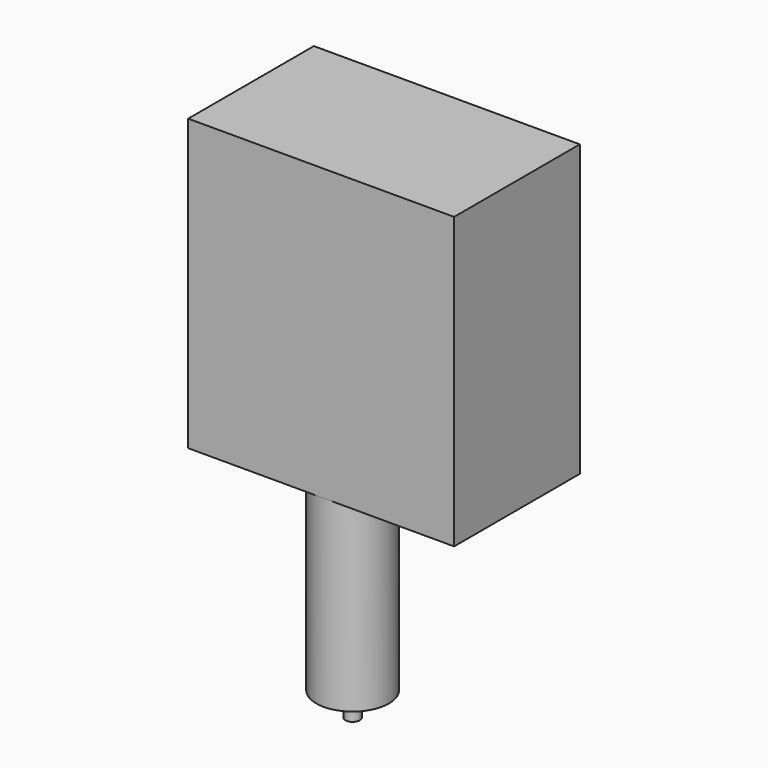
from build123d import *

# Parameters (mm, degrees)
F0_W        = 139.7
F0_H        = 152.4
F1_DEPTH    = 82.55
F2_R        = 19.05
F3_DEPTH    = 96.52
F4_R        = 3.81
F5_DEPTH    = 12.7
F6_T        = 2.54
F6_T4_ANGLE = 270.000000001
F6_T6_ANGLE = 90.000000001


# Not quite as in the source:
# - a shell that OpenCascade refuses in one call is made with other operations: the cavity is built on its own and cut out


with BuildPart() as f1:
    # F0 (on Front) → F1 (new body)
    with BuildSketch(Plane.XZ):
        with Locations((-1.2888036728, 17.3768577993)):
            Rectangle(F0_W, F0_H)
    extrude(amount=-F1_DEPTH)

    # F2 (on face) → F3 (join)
    with BuildSketch(Plane(origin=(0, 0, -58.8231422007), x_dir=(1, 0, 0), z_dir=(0, 0, -1))):
        with Locations((0, -19.05)):
            Circle(F2_R)
    extrude(amount=F3_DEPTH)

    # F4 (on face) → F5 (join)
    with BuildSketch(Plane(origin=(0, 0, -155.3431422007), x_dir=(1, 0, 0), z_dir=(0, 0, -1))):
        with Locations((0, -19.05)):
            Circle(F4_R)
    extrude(amount=F5_DEPTH)

    # F6: shell of thickness 2.54, made by hand


with BuildPart() as f6_core1:
    # F6_t2: copy of F1
    add(f1.part)

    # the walls: a layer under each face that stays
    f6_faces = [f6_core1.faces().sort_by_distance(p)[0] for p in [
        (-1.2888036728, 41.275, 93.5768577993),
        (68.5611963272, 41.275, 17.3768577993),
        (-71.1388036728, 41.275, 17.3768577993),
        (-1.2888036728, 0, 17.3768577993),
        (-1.2888036728, 82.55, 17.3768577993),
        (-1.2888036728, 41.275, -58.8231422007),
        (-19.05, 19.05, -107.0831422007),
        (-12.7, 31.75, -155.3431422007),
        (-3.81, 19.05, -161.6931422007),
    ]]
    thicken(f6_faces, amount=-F6_T, mode=Mode.SUBTRACT)

    # F6_s3 → F6_t4 (revolve, cut)
    with BuildSketch(Plane.YZ):
        Polygon((-0.0254, -58.8485422007), (0, -56.2831422007), (2.54, -56.2831422007), (2.54, -58.8231422007), align=None)
    revolve(axis=Axis((0, 19.05, -58.8231422007), (0, 0, -1)), revolution_arc=F6_T4_ANGLE, mode=Mode.SUBTRACT)

    # F6_s5 → F6_t6 (revolve, cut)
    with BuildSketch(Plane.XZ.offset(-19.05)):
        Polygon((19.0754, -58.8485422007), (19.05, -56.2831422007), (16.51, -56.2831422007), (16.51, -58.8231422007), align=None)
    revolve(axis=Axis((0, 19.05, -58.8231422007), (0, 0, -1)), revolution_arc=F6_T6_ANGLE, mode=Mode.SUBTRACT)

    # F6_s7 → F6_t8 (revolve, cut)
    with BuildSketch(Plane.XZ.offset(-19.05)):
        Polygon((3.8354, -155.3685422007), (3.81, -152.8031422007), (1.27, -152.8031422007), (1.27, -155.3431422007), align=None)
    revolve(axis=Axis((0, 19.05, -155.3431422007), (0, 0, -1)), mode=Mode.SUBTRACT)


with BuildPart() as f1_1:
    add(f1.part)

    # what is left inside the walls is the cavity
    f6_cavity = [f6_core1.part.solids().sort_by_distance(p)[0] for p in [
        (-1.288804, 79.9846, -7.176476),
    ]]
    add(f6_cavity, mode=Mode.SUBTRACT)


solid = f1_1.part
